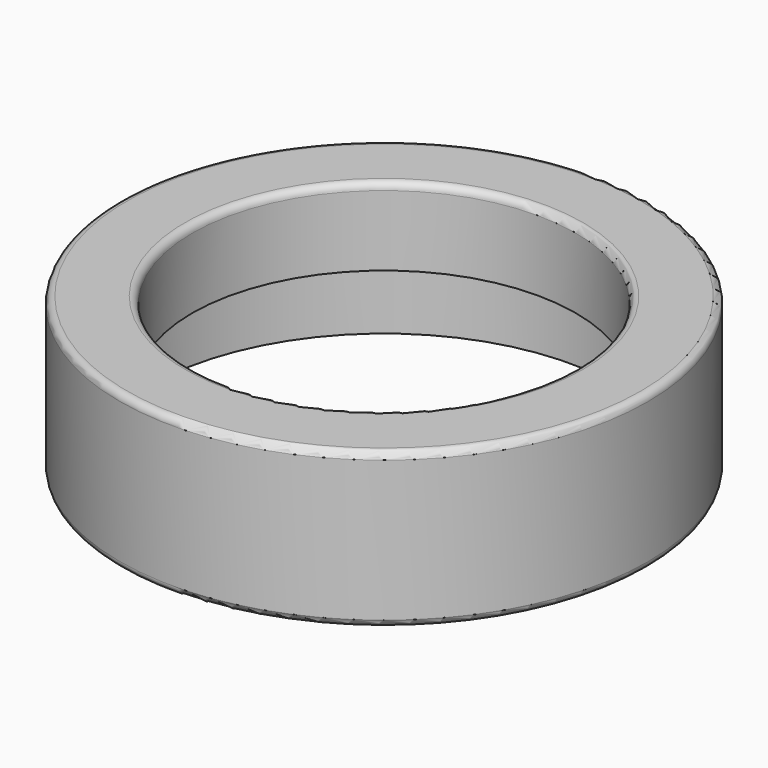
from build123d import *

# Parameters (mm, degrees)
F2_R     = 37.5
F2_R_2   = 33.25
F2_R_3   = 27.25
F3_DEPTH = 22
F4_DEPTH = 11
F5_R     = 1


# Not quite as in the source:
# - a feature of the source that left no trace in its solid (it failed there, or was rolled back) is left out


with BuildPart() as f3:
    # F2 (on Top) → F3 (new body)
    with BuildSketch(Plane.XY):
        Circle(F2_R)
        Circle(F2_R_2, mode=Mode.SUBTRACT)
        Circle(F2_R_2)
        Circle(F2_R_3, mode=Mode.SUBTRACT)
    extrude(amount=F3_DEPTH)

    # F2 (on Top) → F4 (cut)
    with BuildSketch(Plane.XY):
        Circle(F2_R_2)
        Circle(F2_R_3, mode=Mode.SUBTRACT)
    extrude(amount=F4_DEPTH, mode=Mode.SUBTRACT)

    # F5
    f5_edges = [f3.edges().sort_by_distance(p)[0] for p in [
        (-37.5, 0, 22),
        (-27.25, 0, 22),
        (-37.5, 0, 0),
    ]]
    fillet(f5_edges, radius=F5_R)


solid = f3.part
